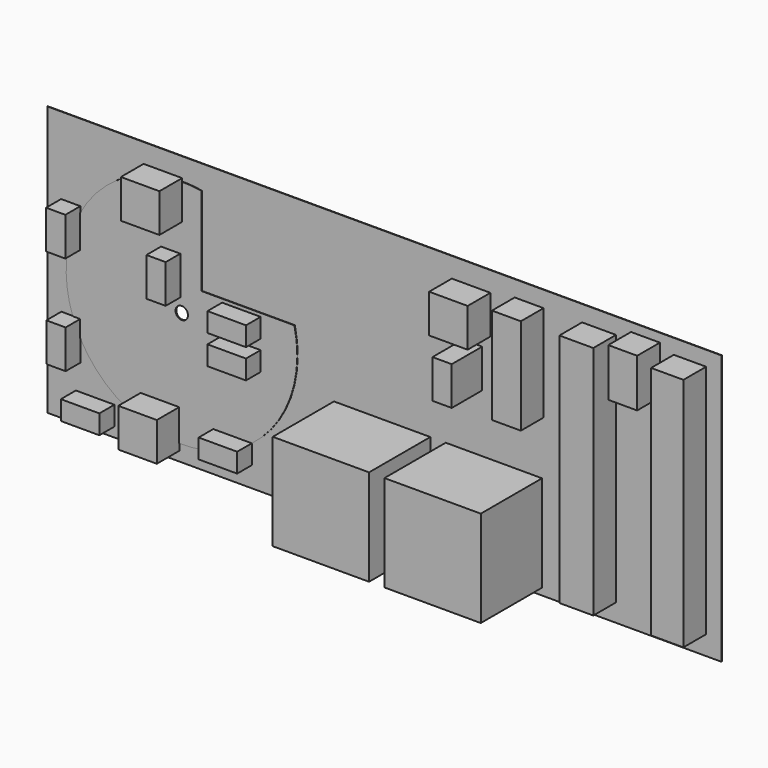
from build123d import *

# Parameters (mm, degrees)
F0_W     = 1677.5682196007
F0_H     = 12225
F1_DEPTH = 1500
F0_W_2   = 1760
F0_W_3   = 1500
F0_H_2   = 5000
F0_H_3   = 2500
F0_W_4   = 2000
F0_H_4   = 1000
F0_W_5   = 5000
F0_W_6   = 1000
F0_H_5   = 2000
F0_W_7   = 4531.0974121094
F0_H_6   = 6739.2702102661
F2_DEPTH = 25
F3_DEPTH = 4000
F4_DEPTH = 1500
F0_R     = 323.2486939486
F5_DEPTH = 50
F6_DEPTH = 2000
F7_DEPTH = 25
F8_DEPTH = 1000


# Not quite as in the source:
# - a feature names something its author has since deleted; it is built from what else it names


with BuildPart() as f1:
    # F0 (on Front) → F1 (new body)
    with BuildSketch(Plane.XZ):
        with Locations((33203.6515982442, -6887.5)):
            Rectangle(F0_W, F0_H)
    extrude(amount=F1_DEPTH)


with BuildPart() as f1b:
    # F0 (on Front) → F1, piece 2 (new body)
    with BuildSketch(Plane.XZ):
        with Locations((28484.8674884439, -6953.9399623871)):
            Rectangle(F0_W_2, F0_H)
    extrude(amount=F1_DEPTH)


with BuildPart() as f1c:
    # F0 (on Front) → F1, piece 3 (new body)
    with BuildSketch(Plane.XZ):
        with Locations((24854.8674884439, -3341.4399623871)):
            Rectangle(F0_W_3, F0_H_2)
    extrude(amount=F1_DEPTH)


with BuildPart() as f1d:
    # F0 (on Front) → F1, piece 4 (new body)
    with BuildSketch(Plane.XZ):
        with Locations((30892.4357080446, -1704.4703960419)):
            Rectangle(F0_W_3, F0_H_3)
    extrude(amount=F1_DEPTH)


with BuildPart() as f2:
    # F0 (on Front) → F2 (new body)
    with BuildSketch(Plane.XZ):
        Polygon((15060.6956481934, 0), (-157.5642919554, 0), (-157.5642919554, -14000), (34842.4357080446, -14000), (34842.4357080446, 0), (19591.7930603027, 0), (19591.7930603027, -6739.2702102661), (15060.6956481934, -6739.2702102661), align=None)
        with Locations((2325.9228467941, -13000)):
            Rectangle(F0_W_4, F0_H_4, mode=Mode.SUBTRACT)
        with Locations((17224.8674884439, -11142.5313949585)):
            Rectangle(F0_W_5, F0_H_2, mode=Mode.SUBTRACT)
        with BuildLine():
            Line((10478.7209733374, -12926.2115996243), (8478.7209733374, -12926.2115996243))
            ThreePointArc((8478.7209733374, -12926.2115996243), (7601.9868729202, -13105.3703999085), (6708.3578109742, -13152.142808433))
            Line((6708.3578109741, -13152.142808433), (6708.3578109741, -13500))
            Line((6708.3578109741, -13500), (4708.3578109741, -13500))
            Line((4708.3578109741, -13500), (4708.3578109741, -12761.2886622132))
            ThreePointArc((4708.3578109742, -12761.2886622131), (2895.3863427984, -11672.5791421162), (1572.7429986001, -10022.497766057))
            Line((1572.7429986, -10022.4977660571), (1572.7429986, -11142.4913406372))
            Line((1572.7429986, -11142.4913406372), (572.7429986, -11142.4913406372))
            Line((572.7429986, -11142.4913406372), (572.7429986, -9142.4913406372))
            Line((572.7429986, -9142.4913406372), (1181.6517873175, -9142.4913406372))
            ThreePointArc((1181.6517873175, -9142.4913406372), (858.0648867062, -7586.4295539984), (954.3874504445, -5999.9999999999))
            Line((954.3874504445, -6000), (559.6692562103, -6000))
            Line((559.6692562103, -6000), (559.6692562103, -4000))
            Line((559.6692562103, -4000), (1559.6692562103, -4000))
            Line((1559.6692562103, -4000), (1559.6692562103, -4308.9304307886))
            ThreePointArc((1559.6692562102, -4308.9304307885), (2939.0128869101, -2596.9657152915), (4842.4357080447, -1496.7868195462))
            Line((4842.4357080446, -1496.7868195462), (4842.4357080446, -1000))
            Line((4842.4357080446, -1000), (6842.4357080446, -1000))
            Line((6842.4357080446, -1000), (6842.4357080446, -1153.6410690386))
            ThreePointArc((6842.4357080447, -1153.6410690386), (7358.9059893254, -1175.9108602927), (7871.5423754885, -1242.5549195207))
            Line((7871.5423754883, -1242.5549195207), (7871.5423754883, -546.0254189148))
            Line((7871.5423754883, -546.0254189148), (13195.7473754883, -546.0254189148))
            Line((13195.7473754883, -546.0254189148), (13195.7473754883, -5818.2864189148))
            Line((13195.7473754883, -5818.2864189148), (12691.9508980747, -5818.2864189148))
            ThreePointArc((12691.9508980747, -5818.2864189149), (12804.695813918, -6481.7374822721), (12842.4357080446, -7153.6410690386))
            ThreePointArc((12842.4357080446, -7153.6410690386), (12219.1313285794, -9816.5613089485), (10478.7209733374, -11926.2115996243))
            Line((10478.7209733374, -11926.2115996243), (10478.7209733374, -12926.2115996243))
        make_face(mode=Mode.SUBTRACT)
        with Locations((23024.8674884439, -11142.5313949585)):
            Rectangle(F0_W_5, F0_H_2, mode=Mode.SUBTRACT)
        with Locations((21917.658996582, -4636.4841461182)):
            Rectangle(F0_W_6, F0_H_5, mode=Mode.SUBTRACT)
        with Locations((28484.8674884439, -6953.9399623871)):
            Rectangle(F0_W_2, F0_H, mode=Mode.SUBTRACT)
        with Locations((33203.6515982442, -6887.5)):
            Rectangle(F0_W, F0_H, mode=Mode.SUBTRACT)
        with Locations((24854.8674884439, -3341.4399623871)):
            Rectangle(F0_W_3, F0_H_2, mode=Mode.SUBTRACT)
        with Locations((21842.4357080446, -2039.3109321594)):
            Rectangle(F0_W_4, F0_H_5, mode=Mode.SUBTRACT)
        with Locations((30892.4357080446, -1704.4703960419)):
            Rectangle(F0_W_3, F0_H_3, mode=Mode.SUBTRACT)
        with Locations((17326.244354248, -3369.6351051331)):
            Rectangle(F0_W_7, F0_H_6)
        with BuildLine():
            Line((7871.5423754883, -5818.2864189148), (12691.9508980747, -5818.2864189148))
            ThreePointArc((12691.9508980747, -5818.2864189149), (10973.1970607696, -2801.9964779865), (7871.5423754885, -1242.5549195207))
            Line((7871.5423754883, -1242.5549195207), (7871.5423754883, -5818.2864189148))
        make_face()
        with BuildLine():
            ThreePointArc((7871.5423754885, -1242.5549195207), (10973.1970607696, -2801.9964779865), (12691.9508980747, -5818.2864189149))
            Line((12691.9508980747, -5818.2864189148), (13195.7473754883, -5818.2864189148))
            Line((13195.7473754883, -5818.2864189148), (13195.7473754883, -546.0254189148))
            Line((13195.7473754883, -546.0254189148), (7871.5423754883, -546.0254189148))
            Line((7871.5423754883, -546.0254189148), (7871.5423754883, -1242.5549195207))
        make_face()
    extrude(amount=F2_DEPTH)

    # F0 (on Front) → F3 (join)
    with BuildSketch(Plane.XZ):
        with Locations((17224.8674884439, -11142.5313949585)):
            Rectangle(F0_W_5, F0_H_2)
        with Locations((23024.8674884439, -11142.5313949585)):
            Rectangle(F0_W_5, F0_H_2)
    extrude(amount=F3_DEPTH)

    # F0 (on Front) → F4 (join)
    with BuildSketch(Plane.XZ):
        with BuildLine():
            Line((6842.4357080446, -3000), (6842.4357080446, -1153.6410690386))
            ThreePointArc((6842.4357080447, -1153.6410690386), (5827.8238356901, -1240.0497111177), (4842.4357080447, -1496.7868195462))
            Line((4842.4357080446, -1496.7868195462), (4842.4357080446, -3000))
            Line((4842.4357080446, -3000), (6842.4357080446, -3000))
        make_face()
        with BuildLine():
            ThreePointArc((4842.4357080447, -1496.7868195462), (5827.8238356901, -1240.0497111177), (6842.4357080447, -1153.6410690386))
            Line((6842.4357080446, -1153.6410690386), (6842.4357080446, -1000))
            Line((6842.4357080446, -1000), (4842.4357080446, -1000))
            Line((4842.4357080446, -1000), (4842.4357080446, -1496.7868195462))
        make_face()
        with BuildLine():
            ThreePointArc((4708.3578109742, -12761.2886622131), (5691.6427564117, -13042.2466410287), (6708.3578109742, -13152.142808433))
            Line((6708.3578109741, -13152.142808433), (6708.3578109741, -11500))
            Line((6708.3578109741, -11500), (4708.3578109741, -11500))
            Line((4708.3578109741, -11500), (4708.3578109741, -12761.2886622132))
        make_face()
        with BuildLine():
            Line((6708.3578109741, -13500), (6708.3578109741, -13152.142808433))
            ThreePointArc((6708.3578109742, -13152.142808433), (5691.6427564117, -13042.2466410287), (4708.3578109742, -12761.2886622131))
            Line((4708.3578109741, -12761.2886622132), (4708.3578109741, -13500))
            Line((4708.3578109741, -13500), (6708.3578109741, -13500))
        make_face()
        with Locations((21842.4357080446, -2039.3109321594)):
            Rectangle(F0_W_4, F0_H_5)
    extrude(amount=F4_DEPTH)

    # F0 (on Front) → F5 (join)
    with BuildSketch(Plane.XZ):
        with BuildLine():
            ThreePointArc((6708.3578109742, -13152.142808433), (7601.9868729202, -13105.3703999085), (8478.7209733374, -12926.2115996243))
            Line((8478.7209733374, -12926.2115996243), (8478.7209733374, -11926.2115996243))
            Line((8478.7209733374, -11926.2115996243), (10478.7209733374, -11926.2115996243))
            ThreePointArc((10478.7209733374, -11926.2115996243), (12219.1313285794, -9816.5613089485), (12842.4357080446, -7153.6410690386))
            ThreePointArc((12842.4357080446, -7153.6410690386), (12804.695813918, -6481.7374822721), (12691.9508980747, -5818.2864189149))
            Line((12691.9508980747, -5818.2864189148), (7871.5423754883, -5818.2864189148))
            Line((7871.5423754883, -5818.2864189148), (7871.5423754883, -1242.5549195207))
            ThreePointArc((7871.5423754885, -1242.5549195207), (7358.9059893254, -1175.9108602927), (6842.4357080447, -1153.6410690386))
            Line((6842.4357080446, -1153.6410690386), (6842.4357080446, -3000))
            Line((6842.4357080446, -3000), (4842.4357080446, -3000))
            Line((4842.4357080446, -3000), (4842.4357080446, -1496.7868195462))
            ThreePointArc((4842.4357080447, -1496.7868195462), (2939.0128869101, -2596.9657152915), (1559.6692562102, -4308.9304307885))
            Line((1559.6692562103, -4308.9304307886), (1559.6692562103, -6000))
            Line((1559.6692562103, -6000), (954.3874504445, -6000))
            ThreePointArc((954.3874504445, -5999.9999999999), (858.0648867062, -7586.4295539984), (1181.6517873175, -9142.4913406372))
            Line((1181.6517873175, -9142.4913406372), (1572.7429986, -9142.4913406372))
            Line((1572.7429986, -9142.4913406372), (1572.7429986, -10022.4977660571))
            ThreePointArc((1572.7429986001, -10022.497766057), (2895.3863427984, -11672.5791421162), (4708.3578109742, -12761.2886622131))
            Line((4708.3578109741, -12761.2886622132), (4708.3578109741, -11500))
            Line((4708.3578109741, -11500), (6708.3578109741, -11500))
            Line((6708.3578109741, -11500), (6708.3578109741, -13152.142808433))
        make_face()
        with Locations((6842.4357080446, -7153.6410690386)):
            Circle(F0_R, mode=Mode.SUBTRACT)
        with Locations((9935.4639053345, -8019.3462371826)):
            Rectangle(F0_W_4, F0_H_4, mode=Mode.SUBTRACT)
        with Locations((6267.0893669128, -5467.5793647766)):
            Rectangle(F0_W_6, F0_H_5, mode=Mode.SUBTRACT)
        with Locations((9936.3832473755, -6500)):
            Rectangle(F0_W_4, F0_H_4, mode=Mode.SUBTRACT)
    extrude(amount=F5_DEPTH)

    # F0 (on Front) → F6 (join)
    with BuildSketch(Plane.XZ):
        with Locations((21917.658996582, -4636.4841461182)):
            Rectangle(F0_W_6, F0_H_5)
    extrude(amount=F6_DEPTH)

    # F0 (on Front) → F7 (join)
    with BuildSketch(Plane.XZ):
        with Locations((9936.3832473755, -6500)):
            Rectangle(F0_W_4, F0_H_4)
    extrude(amount=F7_DEPTH)

    # F0 (on Front) → F8 (join)
    with BuildSketch(Plane.XZ):
        with Locations((6267.0893669128, -5467.5793647766)):
            Rectangle(F0_W_6, F0_H_5)
        with BuildLine():
            Line((559.6692562103, -6000), (954.3874504445, -6000))
            ThreePointArc((954.3874504445, -5999.9999999999), (1193.3911525372, -5131.6876546661), (1559.6692562102, -4308.9304307885))
            Line((1559.6692562103, -4308.9304307886), (1559.6692562103, -4000))
            Line((1559.6692562103, -4000), (559.6692562103, -4000))
            Line((559.6692562103, -4000), (559.6692562103, -6000))
        make_face()
        with BuildLine():
            ThreePointArc((1559.6692562102, -4308.9304307885), (1193.3911525372, -5131.6876546661), (954.3874504445, -5999.9999999999))
            Line((954.3874504445, -6000), (1559.6692562103, -6000))
            Line((1559.6692562103, -6000), (1559.6692562103, -4308.9304307886))
        make_face()
        with BuildLine():
            Line((1572.7429986, -11142.4913406372), (1572.7429986, -10022.4977660571))
            ThreePointArc((1572.7429986001, -10022.497766057), (1359.5137983438, -9590.3534714618), (1181.6517873175, -9142.4913406372))
            Line((1181.6517873175, -9142.4913406372), (572.7429986, -9142.4913406372))
            Line((572.7429986, -9142.4913406372), (572.7429986, -11142.4913406372))
            Line((572.7429986, -11142.4913406372), (1572.7429986, -11142.4913406372))
        make_face()
        with BuildLine():
            ThreePointArc((1181.6517873175, -9142.4913406372), (1359.5137983438, -9590.3534714618), (1572.7429986001, -10022.497766057))
            Line((1572.7429986, -10022.4977660571), (1572.7429986, -9142.4913406372))
            Line((1572.7429986, -9142.4913406372), (1181.6517873175, -9142.4913406372))
        make_face()
        with Locations((2325.9228467941, -13000)):
            Rectangle(F0_W_4, F0_H_4)
        with BuildLine():
            Line((8478.7209733374, -11926.2115996243), (8478.7209733374, -12926.2115996243))
            ThreePointArc((8478.7209733374, -12926.2115996243), (9525.7172810443, -12520.2042150381), (10478.7209733374, -11926.2115996243))
            Line((10478.7209733374, -11926.2115996243), (8478.7209733374, -11926.2115996243))
        make_face()
        with BuildLine():
            ThreePointArc((10478.7209733374, -11926.2115996243), (9525.7172810443, -12520.2042150381), (8478.7209733374, -12926.2115996243))
            Line((8478.7209733374, -12926.2115996243), (10478.7209733374, -12926.2115996243))
            Line((10478.7209733374, -12926.2115996243), (10478.7209733374, -11926.2115996243))
        make_face()
        with Locations((9935.4639053345, -8019.3462371826)):
            Rectangle(F0_W_4, F0_H_4)
        with Locations((9936.3832473755, -6500)):
            Rectangle(F0_W_4, F0_H_4)
    extrude(amount=F8_DEPTH)


solid = Compound([f1.part, f1b.part, f1c.part, f1d.part, f2.part])
